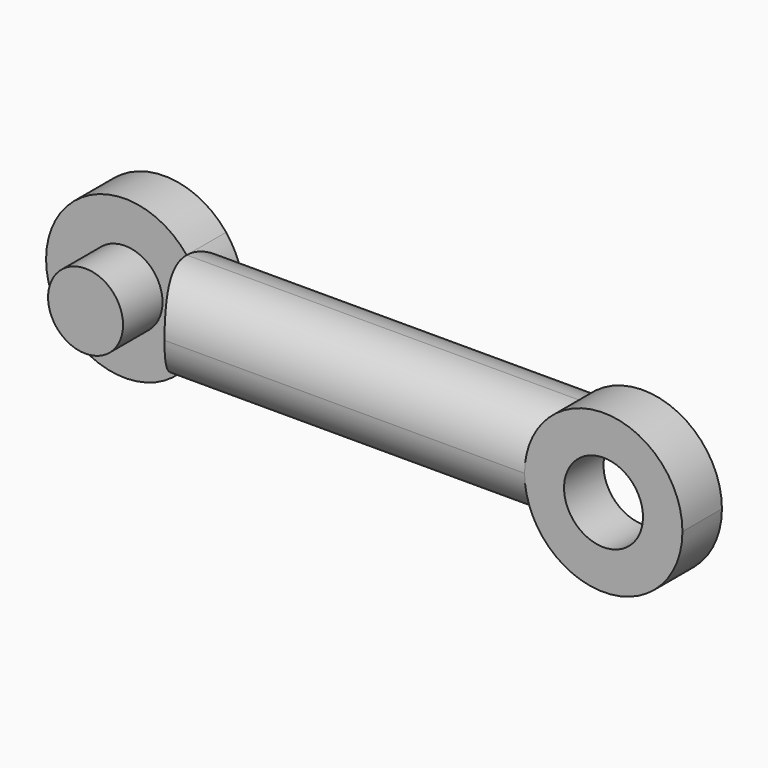
from build123d import *

# Parameters (mm, degrees)
F1_DEPTH = 6.35
F2_R     = 6.3499
F0_R     = 5.08
F3_DEPTH = 6.35
F0_R_2   = 4.826
F4_DEPTH = 6.35
F5_DEPTH = 6.35


# Not quite as in the source:
# - a fillet or chamfer is up to 0.001 mm smaller than in the source, because OpenCascade refuses the exact size


with BuildPart() as f1:
    # F0 (on Front) → F1 (new body, symmetric)
    with BuildSketch(Plane.XZ):
        with BuildLine():
            Line((25.4, 6.35), (-25.4, 6.35))
            ThreePointArc((-25.4, 6.35), (-23.7445407024, 3.3649028089), (-23.171147458, 0))
            ThreePointArc((-23.171147458, 0), (-23.7445407024, -3.3649028089), (-25.4, -6.35))
            Line((-25.4, -6.35), (25.4, -6.35))
            ThreePointArc((25.4, -6.35), (23.171147458, 0), (25.4, 6.35))
        make_face()
    extrude(amount=F1_DEPTH, both=True)

    # F2 (radius 6.35 in the source; OpenCascade refuses exactly that, so slightly less here)
    f2_edges = [f1.edges().sort_by_distance(p)[0] for p in [
        (0, -6.35, 6.35),
        (0, 6.35, 6.35),
        (0, -6.35, -6.35),
        (0, 6.35, -6.35),
    ]]
    fillet(f2_edges, radius=F2_R)

    # F0 (on Front) → F3 (join)
    with BuildSketch(Plane.XZ):
        with BuildLine():
            ThreePointArc((43.491147458, 0), (36.6960502669, 9.5866067556), (25.4, 6.35))
            Line((25.4, 6.35), (25.4, -6.35))
            ThreePointArc((25.4, -6.35), (36.6960502669, -9.5866067556), (43.491147458, 0))
        make_face()
        with Locations((33.331147458, 0)):
            Circle(F0_R, mode=Mode.SUBTRACT)
        with BuildLine():
            Line((25.4, -6.35), (25.4, 6.35))
            ThreePointArc((25.4, 6.35), (23.171147458, 0), (25.4, -6.35))
        make_face()
    extrude(amount=F3_DEPTH)

    # F0 (on Front) → F4 (join)
    with BuildSketch(Plane.XZ):
        with BuildLine():
            Line((-25.4, -6.35), (-25.4, 6.35))
            ThreePointArc((-25.4, 6.35), (-43.491147458, 0), (-25.4, -6.35))
        make_face()
        with Locations((-33.331147458, 0)):
            Circle(F0_R_2, mode=Mode.SUBTRACT)
        with BuildLine():
            ThreePointArc((-23.171147458, 0), (-23.7445407024, 3.3649028089), (-25.4, 6.35))
            Line((-25.4, 6.35), (-25.4, -6.35))
            ThreePointArc((-25.4, -6.35), (-23.7445407024, -3.3649028089), (-23.171147458, 0))
        make_face()
    extrude(amount=-F4_DEPTH)

    # F0 (on Front) → F5 (join, symmetric)
    with BuildSketch(Plane.XZ):
        with Locations((-33.331147458, 0)):
            Circle(F0_R_2)
    extrude(amount=F5_DEPTH, both=True)


solid = f1.part
